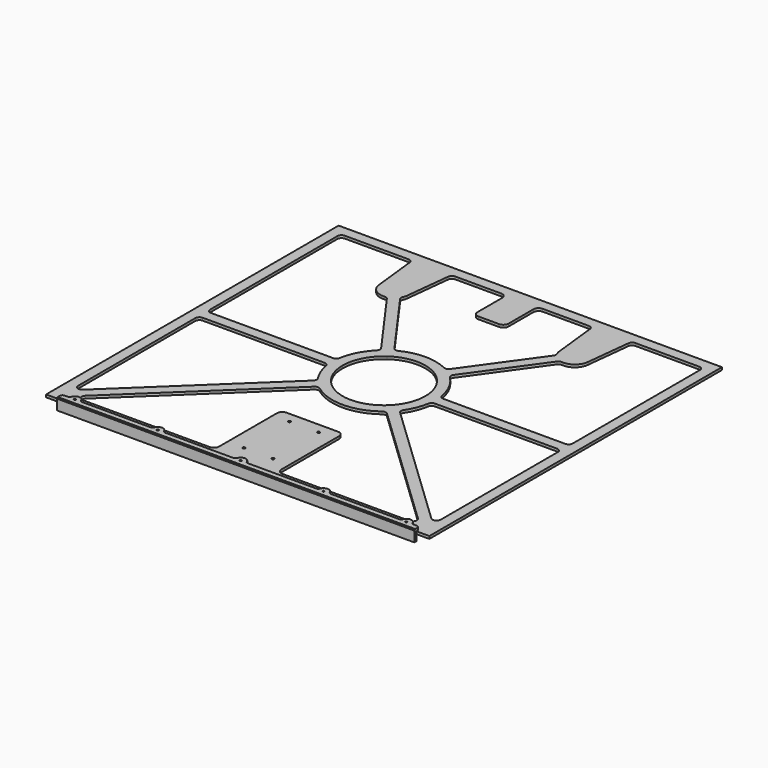
from build123d import *

# Parameters (mm, degrees)
F1_W        = 469.9
F1_H        = 448.31
F2_DEPTH    = 3.175
F5_W        = 15.875
F5_H        = 3.175
F6_DEPTH    = 438.15
F8_DEPTH    = 25.4
F10_D       = 3.048
F10_DEPTH   = 25.4
F10_TIP     = 0.9157115834
F12_DEPTH   = 25.4
F13_D       = 2.3876
F13_DEPTH   = 25.4
F13_TIP     = 0.717307407
F13_2_D     = 2.3876
F13_2_DEPTH = 25.4
F13_2_TIP   = 0.717307407
F14_R       = 3.175
F15_SIZE    = 1.27
F16_W       = 438.15
F16_H       = 5.08
F17_DEPTH   = 25.4


with BuildPart() as f2:
    # F1 (on offset) → F2 (new body)
    with BuildSketch(Plane.XY.offset(3.175)):
        Rectangle(F1_W, F1_H)
    extrude(amount=F2_DEPTH)

    # F7 (on face) → F8 (cut)
    with BuildSketch(Plane.XY.offset(6.35)):
        with BuildLine():
            ThreePointArc((29.5751154163, 41.3031784263), (0, 50.8), (-29.5751154163, 41.3031784263))
            ThreePointArc((-29.5751154163, 41.3031784263), (-45.1832704834, 23.2187869714), (-50.8, 0))
            ThreePointArc((-50.8, 0), (-47.1713277196, -18.8548625338), (-36.8037070406, -35.016098413))
            ThreePointArc((-36.8037070406, -35.016098413), (0, -50.8), (36.8037070406, -35.016098413))
            ThreePointArc((36.8037070406, -35.016098413), (47.1713277196, -18.8548625338), (50.8, 0))
            ThreePointArc((50.8, 0), (45.1832704834, 23.2187869714), (29.5751154163, 41.3031784263))
        make_face()
        with BuildLine():
            ThreePointArc((-217.17, 211.455), (-220.7621024484, 209.9671024484), (-222.25, 206.375))
            Line((-222.25, 206.375), (-222.25, 11.43))
            ThreePointArc((-222.25, 11.43), (-220.7621024484, 7.8378975516), (-217.17, 6.35))
            Line((-217.17, 6.35), (-67.6207919208, 6.35))
            ThreePointArc((-67.6207919208, 6.35), (-64.341666021, 7.5500859116), (-62.6118443711, 10.5833333333))
            ThreePointArc((-62.6118443711, 10.5833333333), (-56.479087955, 29.0234840046), (-45.0566497115, 44.7453720151))
            ThreePointArc((-45.0566497115, 44.7453720151), (-43.5975338397, 47.9177297985), (-44.5308638458, 51.282513318))
            Line((-44.5308638458, 51.282513318), (-104.2050703178, 134.6206292529))
            ThreePointArc((-104.2050703178, 134.6206292529), (-106.2303786696, 136.2864644475), (-108.8166292444, 136.7202717547))
            ThreePointArc((-108.8166292444, 136.7202717547), (-121.642256321, 140.6064593443), (-128.0486868765, 152.377475079))
            Line((-128.0486868765, 152.377475079), (-134.0371794017, 206.9293327319))
            ThreePointArc((-134.0371794017, 206.9293327319), (-135.6963878256, 210.1580153501), (-139.086844264, 211.455))
            Line((-139.086844264, 211.455), (-217.17, 211.455))
        make_face()
        with BuildLine():
            Line((222.25, -190.8449625627), (222.25, -11.4299999233))
            ThreePointArc((222.25, -11.4299999233), (220.7621024484, -7.8378974748), (217.17, -6.3499999233))
            Line((217.17, -6.3499999233), (67.6207919338, -6.3499999233))
            ThreePointArc((67.6207919338, -6.3499999233), (64.3416660318, -7.5500858367), (62.6118443831, -10.5833332623))
            ThreePointArc((62.6118443831, -10.5833332623), (58.9641596629, -23.5685781338), (52.6562011623, -35.4904843465))
            ThreePointArc((52.6562011623, -35.4904843465), (51.8186294892, -38.880373217), (53.367087414, -42.0100937983))
            Line((53.367087414, -42.0100937983), (213.6683901587, -194.5253332668))
            ThreePointArc((213.6683901587, -194.5253332668), (219.1722764552, -195.5137192491), (222.25, -190.8449625627))
        make_face()
        with BuildLine():
            ThreePointArc((-203.8300628881, -202.6946292959), (-205.0455858188, -208.2604862534), (-200.3284530468, -211.455))
            Line((-200.3284530468, -211.455), (-44.45, -211.455))
            ThreePointArc((-44.45, -211.455), (-39.9598719395, -209.5951280605), (-38.1, -205.105))
            Line((-38.1, -205.105), (-38.1, -116.205))
            ThreePointArc((-38.1, -116.205), (-36.2401280605, -111.7148719395), (-31.75, -109.855))
            Line((-31.75, -109.855), (0, -109.855))
            Line((0, -109.855), (31.75, -109.855))
            ThreePointArc((31.75, -109.855), (36.2401280605, -111.7148719395), (38.1, -116.205))
            Line((38.1, -116.205), (38.1, -205.105))
            ThreePointArc((38.1, -205.105), (39.9598719395, -209.5951280605), (44.45, -211.455))
            Line((44.45, -211.455), (200.3284530468, -211.455))
            ThreePointArc((200.3284530468, -211.455), (205.0455858188, -208.2604862534), (203.8300628881, -202.6946292959))
            Line((203.8300628881, -202.6946292959), (44.6130593958, -51.2110231161))
            ThreePointArc((44.6130593958, -51.2110231161), (41.4101793301, -49.82018484), (38.0661569949, -50.8253646483))
            ThreePointArc((38.0661569949, -50.8253646483), (0, -63.5), (-38.0661569949, -50.8253646483))
            ThreePointArc((-38.0661569949, -50.8253646483), (-41.4101793301, -49.82018484), (-44.6130593958, -51.2110231161))
            Line((-44.6130593958, -51.2110231161), (-203.8300628881, -202.6946292959))
        make_face()
        with BuildLine():
            ThreePointArc((-81.893155736, 211.455), (-85.2836121744, 210.1580153501), (-86.9428205983, 206.9293327319))
            Line((-86.9428205983, 206.9293327319), (-92.9313131235, 152.377475079))
            ThreePointArc((-92.9313131235, 152.377475079), (-93.44748902, 149.660039651), (-94.3815523596, 147.0565000336))
            ThreePointArc((-94.3815523596, 147.0565000336), (-94.8039391414, 144.4683598196), (-93.8792765118, 142.0144080308))
            Line((-93.8792765118, 142.0144080308), (-34.2050697361, 58.6762916717))
            ThreePointArc((-34.2050697361, 58.6762916717), (-31.320268762, 56.7088577588), (-27.846992494, 57.0683363087))
            ThreePointArc((-27.846992494, 57.0683363087), (0, 63.5), (27.846992494, 57.0683363087))
            ThreePointArc((27.846992494, 57.0683363087), (31.320268762, 56.7088577588), (34.2050697361, 58.6762916717))
            Line((34.2050697361, 58.6762916717), (93.8792765118, 142.0144080308))
            ThreePointArc((93.8792765118, 142.0144080308), (94.8039391414, 144.4683598196), (94.3815523596, 147.0565000336))
            ThreePointArc((94.3815523596, 147.0565000336), (93.44748902, 149.660039651), (92.9313131235, 152.377475079))
            Line((92.9313131235, 152.377475079), (86.9428205983, 206.9293327319))
            ThreePointArc((86.9428205983, 206.9293327319), (85.2836121744, 210.1580153501), (81.893155736, 211.455))
            Line((81.893155736, 211.455), (25.4, 211.455))
            ThreePointArc((25.4, 211.455), (20.9098719395, 209.5951280605), (19.05, 205.105))
            Line((19.05, 205.105), (19.05, 167.005))
            ThreePointArc((19.05, 167.005), (17.1901280605, 162.5148719395), (12.7, 160.655))
            Line((12.7, 160.655), (-12.7, 160.655))
            ThreePointArc((-12.7, 160.655), (-17.1901280605, 162.5148719395), (-19.05, 167.005))
            Line((-19.05, 167.005), (-19.05, 205.105))
            ThreePointArc((-19.05, 205.105), (-20.9098719395, 209.5951280605), (-25.4, 211.455))
            Line((-25.4, 211.455), (-81.893155736, 211.455))
        make_face()
        with BuildLine():
            ThreePointArc((139.086844264, 211.455), (135.6963878256, 210.1580153501), (134.0371794017, 206.9293327319))
            Line((134.0371794017, 206.9293327319), (128.0486868765, 152.377475079))
            ThreePointArc((128.0486868765, 152.377475079), (121.642256321, 140.6064593443), (108.8166292444, 136.7202717547))
            ThreePointArc((108.8166292444, 136.7202717547), (106.2303786696, 136.2864644475), (104.2050703178, 134.6206292529))
            Line((104.2050703178, 134.6206292529), (44.5308638458, 51.282513318))
            ThreePointArc((44.5308638458, 51.282513318), (43.5975338397, 47.9177297985), (45.0566497115, 44.7453720151))
            ThreePointArc((45.0566497115, 44.7453720151), (56.479087955, 29.0234840046), (62.6118443711, 10.5833333333))
            ThreePointArc((62.6118443711, 10.5833333333), (64.341666021, 7.5500859116), (67.6207919208, 6.35))
            Line((67.6207919208, 6.35), (217.17, 6.35))
            ThreePointArc((217.17, 6.35), (220.7621024484, 7.8378975516), (222.25, 11.43))
            Line((222.25, 11.43), (222.25, 206.375))
            ThreePointArc((222.25, 206.375), (220.7621024484, 209.9671024484), (217.17, 211.455))
            Line((217.17, 211.455), (139.086844264, 211.455))
        make_face()
        with BuildLine():
            ThreePointArc((-52.6562011623, -35.4904843465), (-58.9641596629, -23.5685781338), (-62.6118443831, -10.5833332623))
            ThreePointArc((-62.6118443831, -10.5833332623), (-64.3416660318, -7.5500858367), (-67.6207919338, -6.3499999233))
            Line((-67.6207919338, -6.3499999233), (-217.17, -6.3499999233))
            ThreePointArc((-217.17, -6.3499999233), (-220.7621024484, -7.8378974748), (-222.25, -11.4299999233))
            Line((-222.25, -11.4299999233), (-222.25, -190.8449625627))
            ThreePointArc((-222.25, -190.8449625627), (-219.1722764552, -195.5137192491), (-213.6683901587, -194.5253332668))
            Line((-213.6683901587, -194.5253332668), (-53.367087414, -42.0100937983))
            ThreePointArc((-53.367087414, -42.0100937983), (-51.8186294892, -38.880373217), (-52.6562011623, -35.4904843465))
        make_face()
    extrude(amount=-F8_DEPTH, mode=Mode.SUBTRACT)

    # F10
    with Locations(Plane.XY.offset(6.35)):
        with Locations((-17.78, -122.555), (17.78, -122.555), (17.78, -192.405), (-17.78, -192.405)):
            Hole(F10_D / 2, depth=F10_DEPTH)
            with Locations((0, 0, -(F10_DEPTH + F10_TIP / 2))):  # 118° drill point
                Cone(0, F10_D / 2, F10_TIP, mode=Mode.SUBTRACT)

    # F13
    with Locations(Plane.XY.offset(9.525)):
        with Locations((-203.2, -219.71), (-101.6, -219.71), (0, -219.71), (101.6, -219.71), (203.2, -219.71)):
            Hole(F13_D / 2, depth=F13_DEPTH)
            with Locations((0, 0, -(F13_DEPTH + F13_TIP / 2))):  # 118° drill point
                Cone(0, F13_D / 2, F13_TIP, mode=Mode.SUBTRACT)


with BuildPart() as f6:
    # F5 (on line) → F6 (new body)
    with BuildSketch(Plane.YZ.offset(-219.075)):
        Polygon((-224.155, -9.525), (-224.155, 6.35), (-224.155, 9.525), (-227.33, 9.525), (-227.33, -9.525), align=None)
        with Locations((-216.2175, 7.9375)):
            Rectangle(F5_W, F5_H)
    extrude(amount=F6_DEPTH)

    # F11 (on face) → F12 (cut)
    with BuildSketch(Plane.XY.offset(9.525)):
        Polygon((-219.075, -202.9420733452), (-219.075, -208.28), (219.075, -208.28), (219.075, -202.9420733452), (0, -202.9420733452), align=None)
        with BuildLine():
            Line((-219.075, -208.28), (-219.075, -219.71))
            Line((-219.075, -219.71), (-209.55, -219.71))
            ThreePointArc((-209.55, -219.71), (-203.2, -213.36), (-196.85, -219.71))
            Line((-196.85, -219.71), (-107.95, -219.71))
            ThreePointArc((-107.95, -219.71), (-101.6, -213.36), (-95.25, -219.71))
            Line((-95.25, -219.71), (-6.35, -219.71))
            ThreePointArc((-6.35, -219.71), (0, -213.36), (6.35, -219.71))
            Line((6.35, -219.71), (95.25, -219.71))
            ThreePointArc((95.25, -219.71), (101.6, -213.36), (107.95, -219.71))
            Line((107.95, -219.71), (196.85, -219.71))
            ThreePointArc((196.85, -219.71), (203.2, -213.36), (209.55, -219.71))
            Line((209.55, -219.71), (219.075, -219.71))
            Line((219.075, -219.71), (219.075, -208.28))
            Line((219.075, -208.28), (-219.075, -208.28))
        make_face()
    extrude(amount=-F12_DEPTH, mode=Mode.SUBTRACT)

    # F13#2
    with Locations(Plane.XY.offset(9.525)):
        with Locations((-203.2, -219.71), (-101.6, -219.71), (0, -219.71), (101.6, -219.71), (203.2, -219.71)):
            Hole(F13_2_D / 2, depth=F13_2_DEPTH)
            with Locations((0, 0, -(F13_2_DEPTH + F13_2_TIP / 2))):  # 118° drill point
                Cone(0, F13_2_D / 2, F13_2_TIP, mode=Mode.SUBTRACT)

    # F14
    f14_edges = [f6.edges().sort_by_distance(p)[0] for p in [
        (209.55, -219.71, 7.9375),
        (196.85, -219.71, 7.9375),
        (95.25, -219.71, 7.9375),
        (-6.35, -219.71, 7.9375),
        (6.35, -219.71, 7.9375),
        (107.95, -219.71, 7.9375),
        (-107.95, -219.71, 7.9375),
        (-209.55, -219.71, 7.9375),
        (-95.25, -219.71, 7.9375),
        (-196.85, -219.71, 7.9375),
        (-219.075, -219.71, 7.9375),
        (219.075, -219.71, 7.9375),
    ]]
    fillet(f14_edges, radius=F14_R)

    # F15
    f15_edges = [f6.edges().sort_by_distance(p)[0] for p in [
        (0, -227.33, 9.525),
    ]]
    chamfer(f15_edges, length=F15_SIZE)

    # F16 (on face) → F17 (cut)
    with BuildSketch(Plane.XZ.offset(227.33)):
        with Locations((0, -6.985)):
            Rectangle(F16_W, F16_H)
    extrude(amount=-F17_DEPTH, mode=Mode.SUBTRACT)


solid = Compound([f2.part, f6.part])
